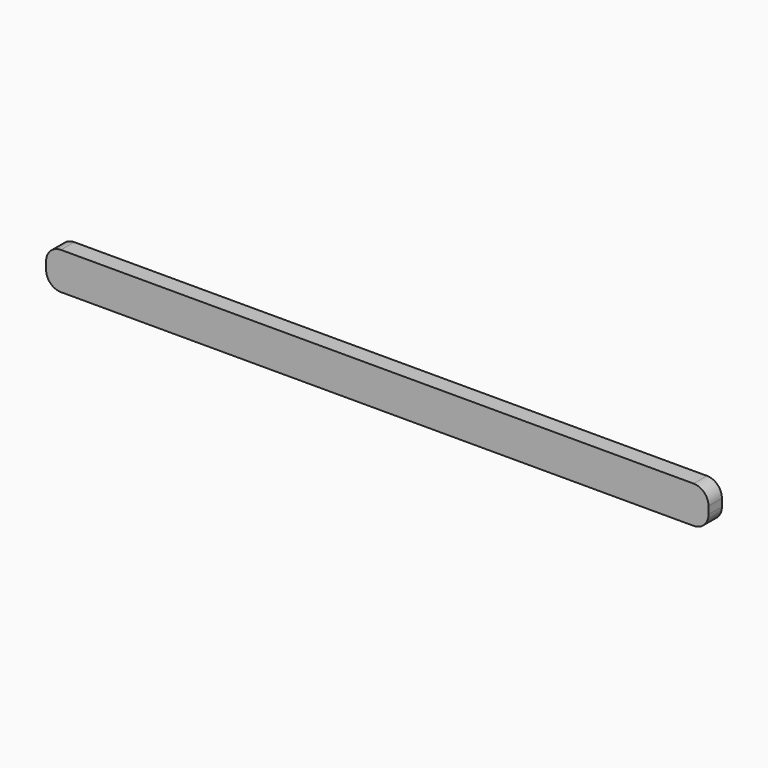
from build123d import *

# Parameters (mm, degrees)
F1_DEPTH = 4.5


# Not quite as in the source:
# - a feature names something its author has since deleted; it is built from what else it names


with BuildPart() as f1:
    # F0 (on Front) → F1 (new body)
    with BuildSketch(Plane.XZ):
        with BuildLine():
            Line((140.551713574, 22.8161337823), (-29.448286426, 22.8161337823))
            ThreePointArc((-29.448286426, 22.8161337823), (-32.2767135507, 21.6445609071), (-33.448286426, 18.8161337823))
            Line((-33.448286426, 18.8161337823), (-33.448286426, 16.8161337823))
            ThreePointArc((-33.448286426, 16.8161337823), (-32.2767135507, 13.9877066576), (-29.448286426, 12.8161337823))
            Line((-29.448286426, 12.8161337823), (140.551713574, 12.8161337823))
            ThreePointArc((140.551713574, 12.8161337823), (143.3801406988, 13.9877066576), (144.551713574, 16.8161337823))
            Line((144.551713574, 16.8161337823), (144.551713574, 18.8161337823))
            ThreePointArc((144.551713574, 18.8161337823), (143.3801406988, 21.6445609071), (140.551713574, 22.8161337823))
        make_face()
    extrude(amount=F1_DEPTH)


solid = f1.part
